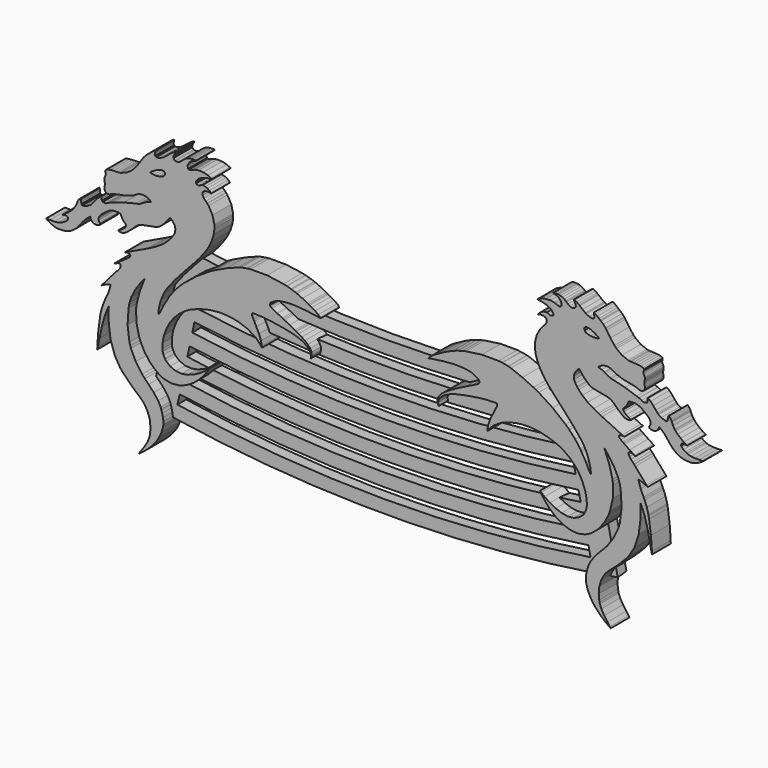
from build123d import *

# Parameters (mm, degrees)
F1_DEPTH               = 3.175
DRAFT_F1_DRAFTED_ANGLE = -3
F3_DEPTH               = 6.35


# Not quite as in the source:
# - an extrude with a draft is written as a straight extrude whose walls are then drafted
# - ends of sketch curves that miss each other by under 0.0002 mm in the source are joined
# - a pattern or mirror of a feature is missing from the dataset's text; its kind, count and spacing are read off the source's solid


with BuildPart() as f1:
    # F0 (on Front) → F1 (new body)
    with BuildSketch(Plane.XZ):
        with BuildLine():
            ThreePointArc((54.301977702, 4.5850323172), (0, 0.5241036), (-54.301977702, 4.5850323172))
            Line((-54.301977702, 4.5850323172), (-63.0060462, -35.368103))
            ThreePointArc((-63.0060462, -35.368103), (0, -40.7508964), (63.0060498531, -35.3681242237))
            Line((63.0060498531, -35.3681242237), (54.301977702, 4.5850323172))
        make_face()
        with BuildLine():
            Line((-56.045319226, -33.2484517718), (-55.3915362015, -30.2474846268))
            ThreePointArc((-55.3915362015, -30.2474846268), (1.30253e-05, -34.4009011827), (55.391562695, -30.2474905326))
            Line((55.391562695, -30.2474905326), (56.0453444328, -33.2484517718))
            ThreePointArc((56.0453444328, -33.2484517718), (1.26034e-05, -37.5759051845), (-56.045319226, -33.2484517718))
        make_face(mode=Mode.SUBTRACT)
        with BuildLine():
            Line((-54.7066751621, -27.1038644939), (-54.0516224279, -24.097069181))
            ThreePointArc((-54.0516224279, -24.097069181), (1.26819e-05, -28.0509044403), (54.051647871, -24.0970702655))
            Line((54.051647871, -24.0970702655), (54.7067017769, -27.103870957))
            ThreePointArc((54.7067017769, -27.103870957), (1.30639e-05, -31.2259008161), (-54.7066751621, -27.1038644939))
        make_face(mode=Mode.SUBTRACT)
        with BuildLine():
            Line((-53.366962814, -20.954373623), (-52.7106531283, -17.9418087047))
            ThreePointArc((-52.7106531283, -17.9418087047), (1.26417e-05, -21.7009048215), (52.710678449, -17.9418092272))
            Line((52.710678449, -17.9418092272), (53.3669877397, -20.9543723325))
            ThreePointArc((53.3669877397, -20.9543723325), (1.25103e-05, -24.875906068), (-53.366962814, -20.954373623))
        make_face(mode=Mode.SUBTRACT)
        with BuildLine():
            Line((-52.0261755137, -14.7999485521), (-51.3686274817, -11.7816994289))
            ThreePointArc((-51.3686274817, -11.7816994289), (1.29118e-05, -15.3509022613), (51.3686535941, -11.7817035856))
            Line((51.3686535941, -11.7817035856), (52.0262007398, -14.7999486408))
            ThreePointArc((52.0262007398, -14.7999486408), (1.26099e-05, -18.525905123), (-52.0261755137, -14.7999485521))
        make_face(mode=Mode.SUBTRACT)
        with BuildLine():
            Line((-50.6843154191, -8.6405991862), (-50.0255472782, -5.6167495712))
            ThreePointArc((-50.0255472782, -5.6167495712), (1.27309e-05, -9.0009039764), (50.0255728549, -5.6167512685))
            Line((50.0255728549, -5.6167512685), (50.6843403575, -8.640597954))
            ThreePointArc((50.6843403575, -8.640597954), (1.25122e-05, -12.1759060495), (-50.6843154191, -8.6405991862))
        make_face(mode=Mode.SUBTRACT)
        with BuildLine():
            Line((-49.3413790575, -2.4763095853), (-48.6814090209, 0.5530569207))
            ThreePointArc((-48.6814090209, 0.5530569207), (1.28477e-05, -2.6509028695), (48.6814349279, 0.5530537068))
            Line((48.6814349279, 0.5530537068), (49.3414053122, -2.4763143953))
            ThreePointArc((49.3414053122, -2.4763143953), (1.29641e-05, -5.8259017661), (-49.3413790575, -2.4763095853))
        make_face(mode=Mode.SUBTRACT)
    extrude(amount=F1_DEPTH)

    # draft_F1_drafted
    draft_f1_drafted_walls = [f1.faces().sort_by_distance(p)[0] for p in [
        (9.199e-07, -2.1166666667, -40.7508964),
        (58.6540137775, -2.1166666667, -15.3915459532),
        (0, -2.1166666667, 0.5241036),
        (-58.654011951, -2.1166666667, -15.3915353414),
        (55.7184535639, -2.1166666667, -31.7479711522),
        (1.26034e-05, -2.1166666667, -37.5759051845),
        (-55.7184277137, -2.1166666667, -31.7479681993),
        (1.30253e-05, -2.1166666667, -34.4009011827),
        (-54.379148795, -2.1166666667, -25.6004668374),
        (1.26819e-05, -2.1166666667, -28.0509044403),
        (54.379174824, -2.1166666667, -25.6004706112),
        (1.30639e-05, -2.1166666667, -31.2259008161),
        (-53.0388079711, -2.1166666667, -19.4480911639),
        (1.26417e-05, -2.1166666667, -21.7009048215),
        (53.0388330943, -2.1166666667, -19.4480907798),
        (1.25103e-05, -2.1166666667, -24.875906068),
        (-51.6974014977, -2.1166666667, -13.2908239905),
        (1.29118e-05, -2.1166666667, -15.3509022613),
        (51.697427167, -2.1166666667, -13.2908261132),
        (1.26099e-05, -2.1166666667, -18.525905123),
        (-50.3549313487, -2.1166666667, -7.1286743787),
        (1.27309e-05, -2.1166666667, -9.0009039764),
        (50.3549566062, -2.1166666667, -7.1286746113),
        (1.25122e-05, -2.1166666667, -12.1759060495),
        (-49.0113940392, -2.1166666667, -0.9616263323),
        (1.28477e-05, -2.1166666667, -2.6509028695),
        (49.0114201201, -2.1166666667, -0.9616303443),
        (1.29641e-05, -2.1166666667, -5.8259017661),
    ]]
    draft(draft_f1_drafted_walls, neutral_plane=Plane.XZ, angle=DRAFT_F1_DRAFTED_ANGLE)

    # F2 (on Front) → F3 (join)
    with BuildSketch(Plane.XZ):
        with BuildLine():
            Line((68.4158652, 8.8282272), (68.6661822, 9.411335))
            ThreePointArc((68.6661822, 9.411335), (70.4497514451, 9.5479214977), (72.1365475574, 8.9525417468))
            Line((72.1365475574, 8.9525417468), (72.3567006, 8.7865712))
            Line((72.3567006, 8.7865712), (72.4553542, 8.712581))
            Line((72.4553542, 8.712581), (72.7564712, 8.4946236))
            Line((72.7564712, 8.4946236), (73.2147634, 8.1538318))
            Line((73.2147634, 8.1538318), (73.6795326, 7.7712062))
            Line((73.6795326, 7.7712062), (74.1016552, 7.3527666))
            Line((74.1016552, 7.3527666), (74.4297724, 6.9043296))
            Line((74.4297724, 6.9043296), (74.6142526, 6.4323722))
            Line((74.6142526, 6.4323722), (74.6052356, 5.9422792))
            Line((74.6052356, 5.9422792), (74.4351064, 5.5500016))
            Line((74.4351064, 5.5500016), (74.3511086, 5.4405022))
            Line((74.3511086, 5.4405022), (74.3087922, 5.38734))
            Line((74.3087922, 5.38734), (74.2272836, 5.1891946))
            Line((74.2272836, 5.1891946), (74.2681268, 4.9929034))
            Line((74.2681268, 4.9929034), (74.4351064, 4.8472598))
            Line((74.4351064, 4.8472598), (74.6910622, 4.7470822))
            Line((74.6910622, 4.7470822), (74.9957098, 4.6882812))
            Line((74.9957098, 4.6882812), (75.3129812, 4.665599))
            Line((75.3129812, 4.665599), (75.602465, 4.6737778))
            Line((75.602465, 4.6737778), (75.7734324, 4.6935898))
            Line((75.7734324, 4.6935898), (75.8284234, 4.707255))
            Line((75.8284234, 4.707255), (75.932411, 4.734433))
            Line((75.932411, 4.734433), (76.2253746, 4.902581))
            Line((76.2253746, 4.902581), (76.5554984, 5.235194))
            Line((76.5554984, 5.235194), (76.7814568, 5.6511444))
            Line((76.7814568, 5.6511444), (76.8672834, 5.9849258))
            Line((76.8672834, 5.9849258), (76.8699504, 6.0960762))
            Line((76.8699504, 6.0960762), (77.0734298, 5.9551062))
            Line((77.0734298, 5.9551062), (77.6601952, 5.495671))
            Line((77.6601952, 5.495671), (78.3445982, 4.8590708))
            Line((78.3445982, 4.8590708), (78.957678, 4.1556686))
            Line((78.957678, 4.1556686), (79.4008064, 3.5590734))
            Line((79.4008064, 3.5590734), (79.537941, 3.3527746))
            Line((79.537941, 3.3527746), (79.6972498, 3.1141416))
            Line((79.6972498, 3.1141416), (80.6871386, 2.0456144))
            Line((80.6871386, 2.0456144), (81.8571642, 1.1738864))
            Line((81.8571642, 1.1738864), (82.1066176, 1.0330688))
            Line((82.1066176, 1.0330688), (82.3129164, 0.9172448))
            Line((82.3129164, 0.9172448), (82.977355, 0.6477762))
            Line((82.977355, 0.6477762), (83.837907, 0.4498086))
            Line((83.837907, 0.4498086), (84.7266276, 0.3784854))
            Line((84.7266276, 0.3784854), (85.4408502, 0.367665))
            Line((85.4408502, 0.367665), (85.6798388, 0.367665))
            Line((85.6798388, 0.367665), (85.8596454, 0.367665))
            Line((85.8596454, 0.367665), (86.3993954, 0.5149596))
            Line((86.3993954, 0.5149596), (87.341456, 0.8784336))
            Line((87.341456, 0.8784336), (88.2373394, 1.341374))
            Line((88.2373394, 1.341374), (88.7067822, 1.6533114))
            Line((88.7067822, 1.6533114), (88.8187708, 1.7851374))
            Line((88.8187708, 1.7851374), (88.5521216, 1.792478))
            Line((88.5521216, 1.792478), (87.7500658, 1.7734788))
            Line((87.7500658, 1.7734788), (86.6028748, 1.7634712))
            Line((86.6028748, 1.7634712), (85.4798646, 1.8737834))
            Line((85.4798646, 1.8737834), (84.7096096, 2.0934426))
            Line((84.7096096, 2.0934426), (84.4836512, 2.220087))
            Line((84.4836512, 2.220087), (84.376006, 2.2807422))
            Line((84.376006, 2.2807422), (84.0531974, 2.4558752))
            Line((84.0531974, 2.4558752), (83.5351136, 2.7788362))
            Line((83.5351136, 2.7788362), (83.0911724, 3.170301))
            Line((83.0911724, 3.170301), (82.8950082, 3.495929))
            Line((82.8950082, 3.495929), (82.8878454, 3.6079176))
            Line((82.8878454, 3.6079176), (82.8825114, 3.6847272))
            Line((82.8825114, 3.6847272), (82.9176904, 3.9180262))
            Line((82.9176904, 3.9180262), (83.0433442, 4.1068498))
            Line((83.0433442, 4.1068498), (83.2403212, 4.1993312))
            Line((83.2403212, 4.1993312), (83.4854566, 4.2181526))
            Line((83.4854566, 4.2181526), (83.7547474, 4.188333))
            Line((83.7547474, 4.188333), (84.0260448, 4.133342))
            Line((84.0260448, 4.133342), (84.2746854, 4.076192))
            Line((84.2746854, 4.076192), (84.427314, 4.0465248))
            Line((84.427314, 4.0465248), (84.4789776, 4.0418512))
            Line((84.4789776, 4.0418512), (84.257515, 4.1901618))
            Line((84.257515, 4.1901618), (83.59394, 4.6322742))
            Line((83.59394, 4.6322742), (82.7385442, 5.2470304))
            Line((82.7385442, 5.2470304), (81.9439814, 5.9277758))
            Line((81.9439814, 5.9277758), (81.4005484, 6.5073784))
            Line((81.4005484, 6.5073784), (81.2432208, 6.7171824))
            Line((81.2432208, 6.7171824), (81.1339246, 6.862826))
            Line((81.1339246, 6.862826), (80.7036232, 7.5662282))
            Line((80.7036232, 7.5662282), (80.3853358, 8.321802))
            Line((80.3853358, 8.321802), (80.3328594, 8.492617))
            Line((80.3328594, 8.492617), (80.320007, 8.5324442))
            Line((80.320007, 8.5324442), (80.2668448, 8.6465918))
            Line((80.2668448, 8.6465918), (80.1520368, 8.8535764))
            Line((80.1520368, 8.8535764), (80.0045644, 9.0797126))
            Line((80.0045644, 9.0797126), (79.8419028, 9.2903548))
            Line((79.8419028, 9.2903548), (79.6790888, 9.4501716))
            Line((79.6790888, 9.4501716), (79.532607, 9.5251524))
            Line((79.532607, 9.5251524), (79.4206438, 9.479153))
            Line((79.4206438, 9.479153), (79.3634684, 9.3300042))
            Line((79.3634684, 9.3300042), (79.3581344, 9.2785184))
            Line((79.3581344, 9.2785184), (79.3438088, 9.1528646))
            Line((79.3438088, 9.1528646), (79.3309818, 8.7704168))
            Line((79.3309818, 8.7704168), (79.2659832, 8.3238086))
            Line((79.2659832, 8.3238086), (79.0208478, 8.0633316))
            Line((79.0208478, 8.0633316), (78.58506, 8.0715104))
            Line((78.58506, 8.0715104), (78.4530816, 8.1131664))
            Line((78.4530816, 8.1131664), (78.3029422, 8.1609946))
            Line((78.3029422, 8.1609946), (77.496543, 8.4711286))
            Line((77.496543, 8.4711286), (76.7696458, 8.9150698))
            Line((76.7696458, 8.9150698), (76.6603242, 9.0298778))
            Line((76.6603242, 9.0298778), (76.4919984, 9.2053664))
            Line((76.4919984, 9.2053664), (76.0292358, 9.768459))
            Line((76.0292358, 9.768459), (75.336654, 10.6211878))
            Line((75.336654, 10.6211878), (74.5980728, 11.405743))
            Line((74.5980728, 11.405743), (74.0409746, 11.846179))
            Line((74.0409746, 11.846179), (73.8321866, 11.9401844))
            Line((73.8321866, 11.9401844), (73.8276908, 11.7873526))
            Line((73.8276908, 11.7873526), (73.8241856, 11.327257))
            Line((73.8241856, 11.327257), (73.751694, 10.9139736))
            Line((73.751694, 10.9139736), (73.4887278, 10.6825034))
            Line((73.4887278, 10.6825034), (73.0519494, 10.6093514))
            Line((73.0519494, 10.6093514), (72.9072964, 10.6093514))
            Line((72.9072964, 10.6093514), (72.7184982, 10.6093514))
            Line((72.7184982, 10.6093514), (72.1513924, 10.8426504))
            Line((72.1513924, 10.8426504), (71.5494632, 11.1581184))
            Line((71.5494632, 11.1581184), (71.423657, 11.1997744))
            Line((71.423657, 11.1997744), (70.809739, 11.4050826))
            Line((70.809739, 11.4050826), (67.7077894, 12.4300996))
            Line((67.7077894, 12.4300996), (64.5488676, 13.229336))
            Line((64.5488676, 13.229336), (63.9069588, 13.3208268))
            Line((63.9069588, 13.3208268), (63.8001264, 13.3359906))
            Line((63.8001264, 13.3359906), (63.4918466, 13.4644892))
            Line((63.4918466, 13.4644892), (63.0263916, 13.7292842))
            Line((63.0263916, 13.7292842), (62.5634512, 14.0232384))
            Line((62.5634512, 14.0232384), (62.2596672, 14.2058898))
            Line((62.2596672, 14.2058898), (62.1538508, 14.2555468))
            Line((62.1538508, 14.2555468), (62.0300258, 14.313535))
            Line((62.0300258, 14.313535), (61.405262, 14.6218402))
            Line((61.405262, 14.6218402), (60.7561904, 14.8551392))
            Line((60.7561904, 14.8551392), (60.6213672, 14.8759672))
            Line((60.6213672, 14.8759672), (60.5907094, 14.8803106))
            Line((60.5907094, 14.8803106), (60.505721, 14.938121))
            Line((60.505721, 14.938121), (60.5498662, 15.0476204))
            Line((60.5498662, 15.0476204), (60.7118674, 15.1885904))
            Line((60.7118674, 15.1885904), (60.9486716, 15.3440638))
            Line((60.9486716, 15.3440638), (61.219969, 15.4978862))
            Line((61.219969, 15.4978862), (61.4812588, 15.6325316))
            Line((61.4812588, 15.6325316), (61.6927392, 15.7311852))
            Line((61.6927392, 15.7311852), (61.780547, 15.7700218))
            Line((61.780547, 15.7700218), (61.8113826, 15.7771846))
            Line((61.8113826, 15.7771846), (61.9750348, 15.8188406))
            Line((61.9750348, 15.8188406), (62.7324374, 15.9056578))
            Line((62.7324374, 15.9056578), (63.489332, 15.8188406))
            Line((63.489332, 15.8188406), (63.6536446, 15.7728412))
            Line((63.6536446, 15.7728412), (63.8048, 15.7301946))
            Line((63.8048, 15.7301946), (64.4963658, 15.360396))
            Line((64.4963658, 15.360396), (65.1771112, 14.953615))
            Line((65.1771112, 14.953615), (65.323593, 14.8929598))
            Line((65.323593, 14.8929598), (65.4764248, 14.8296376))
            Line((65.4764248, 14.8296376), (67.0170618, 14.2673832))
            Line((67.0170618, 14.2673832), (67.1780216, 14.2257272))
            Line((67.1780216, 14.2257272), (67.4753286, 14.1488922))
            Line((67.4753286, 14.1488922), (69.0124604, 13.8775948))
            Line((69.0124604, 13.8775948), (70.5331076, 13.5494776))
            Line((70.5331076, 13.5494776), (70.8234042, 13.4446518))
            Line((70.8234042, 13.4446518), (70.9318876, 13.4056628))
            Line((70.9318876, 13.4056628), (71.250175, 13.2628386))
            Line((71.250175, 13.2628386), (71.701279, 13.0893566))
            Line((71.701279, 13.0893566), (72.1614, 13.0348736))
            Line((72.1614, 13.0348736), (72.5221816, 13.1435094))
            Line((72.5221816, 13.1435094), (72.6171776, 13.2131816))
            Line((72.6171776, 13.2131816), (72.7001594, 13.2756656))
            Line((72.7001594, 13.2756656), (72.896476, 13.534136))
            Line((72.896476, 13.534136), (73.0402908, 13.9364212))
            Line((73.0402908, 13.9364212), (73.0611188, 14.365859))
            Line((73.0611188, 14.365859), (73.0084392, 14.670659))
            Line((73.0084392, 14.670659), (72.9724474, 14.764639))
            Line((72.9724474, 14.764639), (72.9326202, 14.867636))
            Line((72.9326202, 14.867636), (72.9101412, 15.214092))
            Line((72.9101412, 15.214092), (72.9814644, 15.673197))
            Line((72.9814644, 15.673197), (73.0682816, 16.1299652))
            Line((73.0682816, 16.1299652), (73.0772732, 16.4652706))
            Line((73.0772732, 16.4652706), (73.0511112, 16.5692582))
            Line((73.0511112, 16.5692582), (73.0249492, 16.6722298))
            Line((73.0249492, 16.6722298), (72.891142, 16.9670222))
            Line((72.891142, 16.9670222), (72.725661, 17.2871638))
            Line((72.725661, 17.2871638), (72.656827, 17.6316132))
            Line((72.656827, 17.6316132), (72.7391484, 17.9940712))
            Line((72.7391484, 17.9940712), (72.7906342, 18.1025546))
            Line((72.7906342, 18.1025546), (72.8268038, 18.1803802))
            Line((72.8268038, 18.1803802), (72.8042994, 18.4749948))
            Line((72.8042994, 18.4749948), (72.5013536, 18.735294))
            Line((72.5013536, 18.735294), (71.968741, 18.9046104))
            Line((71.968741, 18.9046104), (71.2953362, 19.0041022))
            Line((71.2953362, 19.0041022), (70.5682612, 19.0545974))
            Line((70.5682612, 19.0545974), (69.8758572, 19.0780924))
            Line((69.8758572, 19.0780924), (69.3052462, 19.0944246))
            Line((69.3052462, 19.0944246), (69.0332884, 19.108928))
            Line((69.0332884, 19.108928), (68.9464712, 19.1260984))
            Line((68.9464712, 19.1260984), (68.571364, 19.2037462))
            Line((68.571364, 19.2037462), (66.8724088, 19.8726552))
            Line((66.8724088, 19.8726552), (65.3895822, 20.9478626))
            Line((65.3895822, 20.9478626), (65.1237966, 21.227161))
            Line((65.1237966, 21.227161), (64.8688314, 21.4947754))
            Line((64.8688314, 21.4947754), (63.7569718, 22.9667562))
            Line((63.7569718, 22.9667562), (62.7244364, 24.501729))
            Line((62.7244364, 24.501729), (62.5101366, 24.8003568))
            Line((62.5101366, 24.8003568), (62.4124736, 24.935688))
            Line((62.4124736, 24.935688), (61.8373922, 25.567767))
            Line((61.8373922, 25.567767), (61.1919528, 26.129361))
            Line((61.1919528, 26.129361), (61.059822, 26.2295132))
            Line((61.059822, 26.2295132), (60.9531674, 26.3101582))
            Line((60.9531674, 26.3101582), (60.6522028, 26.5741404))
            Line((60.6522028, 26.5741404), (60.1910912, 26.9774162))
            Line((60.1910912, 26.9774162), (59.710828, 27.3335496))
            Line((59.710828, 27.3335496), (59.3712046, 27.5106892))
            Line((59.3712046, 27.5106892), (59.250707, 27.5341842))
            Line((59.250707, 27.5341842), (59.2470494, 27.4293584))
            Line((59.2470494, 27.4293584), (59.3213698, 27.1120616))
            Line((59.3213698, 27.1120616), (59.4251796, 26.6292838))
            Line((59.4251796, 26.6292838), (59.3647022, 26.2205216))
            Line((59.3647022, 26.2205216), (59.051063, 26.0298692))
            Line((59.051063, 26.0298692), (58.9434178, 26.0217158))
            Line((58.9434178, 26.0217158), (58.7689452, 26.0098794))
            Line((58.7689452, 26.0098794), (57.9815452, 26.1716774))
            Line((57.9815452, 26.1716774), (57.253632, 26.5442954))
            Line((57.253632, 26.5442954), (57.1098172, 26.6372848))
            Line((57.1098172, 26.6372848), (56.952515, 26.7387832))
            Line((56.952515, 26.7387832), (56.2157626, 27.3118834))
            Line((56.2157626, 27.3118834), (55.4950376, 27.9066244))
            Line((55.4950376, 27.9066244), (55.3458888, 28.0179526))
            Line((55.3458888, 28.0179526), (55.2653962, 28.0786078))
            Line((55.2653962, 28.0786078), (55.0149268, 28.2612592))
            Line((55.0149268, 28.2612592), (54.5766498, 28.5530544))
            Line((54.5766498, 28.5530544), (54.1308544, 28.78201))
            Line((54.1308544, 28.78201), (53.8603952, 28.8570162))
            Line((53.8603952, 28.8570162), (53.7827474, 28.8361882))
            Line((53.7827474, 28.8361882), (53.8505654, 28.7015428))
            Line((53.8505654, 28.7015428), (54.0971994, 28.3162502))
            Line((54.0971994, 28.3162502), (54.3731704, 27.8026368))
            Line((54.3731704, 27.8026368), (54.3893248, 27.3137122))
            Line((54.3893248, 27.3137122), (54.0630364, 26.9419324))
            Line((54.0630364, 26.9419324), (53.9274004, 26.868755))
            Line((53.9274004, 26.868755), (53.7979112, 26.8000988))
            Line((53.7979112, 26.8000988), (53.3259792, 26.7477748))
            Line((53.3259792, 26.7477748), (52.7620484, 26.9474188))
            Line((52.7620484, 26.9474188), (52.2456156, 27.3255486))
            Line((52.2456156, 27.3255486), (51.9013186, 27.6346666))
            Line((51.9013186, 27.6346666), (51.7865106, 27.7368254))
            Line((51.7865106, 27.7368254), (51.6670036, 27.842464))
            Line((51.6670036, 27.842464), (51.2874006, 28.1327606))
            Line((51.2874006, 28.1327606), (50.7837948, 28.4220666))
            Line((50.7837948, 28.4220666), (50.235866, 28.6183832))
            Line((50.235866, 28.6183832), (49.7674138, 28.7150302))
            Line((49.7674138, 28.7150302), (49.6102894, 28.7322006))
            Line((49.6102894, 28.7322006), (49.5577876, 28.7385252))
            Line((49.5577876, 28.7385252), (49.3234726, 28.7556956))
            Line((49.3234726, 28.7556956), (48.8933744, 28.7711896))
            Line((48.8933744, 28.7711896), (48.4900986, 28.7493456))
            Line((48.4900986, 28.7493456), (48.2984556, 28.698698))
            Line((48.2984556, 28.698698), (48.285781, 28.6625284))
            Line((48.285781, 28.6625284), (48.2794564, 28.6482028))
            Line((48.2794564, 28.6482028), (48.3805992, 28.5577026))
            Line((48.3805992, 28.5577026), (48.6518966, 28.4708854))
            Line((48.6518966, 28.4708854), (48.9501942, 28.4102302))
            Line((48.9501942, 28.4102302), (49.1066836, 28.3850588))
            Line((49.1066836, 28.3850588), (49.1300008, 28.3822394))
            Line((49.1300008, 28.3822394), (49.2484918, 28.3695648))
            Line((49.2484918, 28.3695648), (49.5876072, 28.1769312))
            Line((49.5876072, 28.1769312), (50.04689, 27.7439882))
            Line((50.04689, 27.7439882), (50.4005088, 27.2187162))
            Line((50.4005088, 27.2187162), (50.542317, 26.856944))
            Line((50.542317, 26.856944), (50.542317, 26.7359384))
            Line((50.542317, 26.7359384), (50.542317, 26.6372848))
            Line((50.542317, 26.6372848), (50.5024898, 26.341832))
            Line((50.5024898, 26.341832), (50.3905012, 26.0966966))
            Line((50.3905012, 26.0966966), (50.2170446, 25.9747004))
            Line((50.2170446, 25.9747004), (49.9909084, 25.9538724))
            Line((49.9909084, 25.9538724), (49.7224304, 26.0080506))
            Line((49.7224304, 26.0080506), (49.4221262, 26.112851))
            Line((49.4221262, 26.112851), (49.1005114, 26.2460232))
            Line((49.1005114, 26.2460232), (48.850042, 26.3489948))
            Line((48.850042, 26.3489948), (48.76673, 26.3806686))
            Line((48.76673, 26.3806686), (48.4872538, 26.4873232))
            Line((48.4872538, 26.4873232), (47.5823788, 26.635456))
            Line((47.5823788, 26.635456), (46.3065368, 26.5848084))
            Line((46.3065368, 26.5848084), (45.063537, 26.264997))
            Line((45.063537, 26.264997), (44.2253116, 25.8813808))
            Line((44.2253116, 25.8813808), (43.9749946, 25.7115818))
            Line((43.9749946, 25.7115818), (44.2779658, 25.682575))
            Line((44.2779658, 25.682575), (45.1828408, 25.5532636))
            Line((45.1828408, 25.5532636), (46.532673, 25.2069854))
            Line((46.532673, 25.2069854), (47.6971868, 24.57323))
            Line((47.6971868, 24.57323), (48.285781, 23.8309912))
            Line((48.285781, 23.8309912), (48.3497636, 23.552531))
            Line((48.3497636, 23.552531), (48.362616, 23.4956858))
            Line((48.362616, 23.4956858), (48.2894386, 23.2965498))
            Line((48.2894386, 23.2965498), (48.047148, 23.1257348))
            Line((48.047148, 23.1257348), (47.737014, 23.0354124))
            Line((47.737014, 23.0354124), (47.5388686, 23.0137462))
            Line((47.5388686, 23.0137462), (47.4757242, 23.0209344))
            Line((47.4757242, 23.0209344), (47.3907358, 23.0309166))
            Line((47.3907358, 23.0309166), (47.001938, 23.2595674))
            Line((47.001938, 23.2595674), (46.5814918, 23.4566968))
            Line((46.5814918, 23.4566968), (46.4811872, 23.4501944))
            Line((46.4811872, 23.4501944), (46.2975452, 23.4395264))
            Line((46.2975452, 23.4395264), (45.7524358, 23.3482134))
            Line((45.7524358, 23.3482134), (45.1773544, 23.124922))
            Line((45.1773544, 23.124922), (44.6782444, 22.7559616))
            Line((44.6782444, 22.7559616), (44.2941202, 22.3536764))
            Line((44.2941202, 22.3536764), (44.1774834, 22.2108522))
            Line((44.1774834, 22.2108522), (44.3211204, 22.2615252))
            Line((44.3211204, 22.2615252), (44.776898, 22.3465136))
            Line((44.776898, 22.3465136), (45.49648, 22.3601788))
            Line((45.49648, 22.3601788), (46.1410558, 22.1620334))
            Line((46.1410558, 22.1620334), (46.4791806, 21.7985848))
            Line((46.4791806, 21.7985848), (46.5146644, 21.657437))
            Line((46.5146644, 21.657437), (46.5516722, 21.5092788))
            Line((46.5516722, 21.5092788), (46.4791806, 21.0165188))
            Line((46.4791806, 21.0165188), (46.1395572, 20.4469238))
            Line((46.1395572, 20.4469238), (45.6576176, 19.9298306))
            Line((45.6576176, 19.9298306), (45.301154, 19.5735194))
            Line((45.301154, 19.5735194), (45.193839, 19.445224))
            Line((45.193839, 19.445224), (44.8960494, 19.0944246))
            Line((44.8960494, 19.0944246), (43.829351, 17.213834))
            Line((43.829351, 17.213834), (43.3347368, 15.1082756))
            Line((43.3347368, 15.1082756), (43.3240942, 14.6453352))
            Line((43.3240942, 14.6453352), (43.3122578, 14.1642338))
            Line((43.3122578, 14.1642338), (43.5012338, 12.7140716))
            Line((43.5012338, 12.7140716), (44.0716416, 10.8659676))
            Line((44.0716416, 10.8659676), (44.9567046, 9.0987118))
            Line((44.9567046, 9.0987118), (46.078902, 7.411593))
            Line((46.078902, 7.411593), (47.3562426, 5.8012838))
            Line((47.3562426, 5.8012838), (48.7115612, 4.2679874))
            Line((48.7115612, 4.2679874), (50.0658892, 2.8086812))
            Line((50.0658892, 2.8086812), (51.0260854, 1.7734788))
            Line((51.0260854, 1.7734788), (51.3397246, 1.4226794))
            Line((51.3397246, 1.4226794), (51.763676, 0.9489186))
            Line((51.763676, 0.9489186), (53.8369002, -1.3692886))
            Line((53.8369002, -1.3692886), (55.78983, -3.7839904))
            Line((55.78983, -3.7839904), (56.1551074, -4.307586))
            Line((56.1551074, -4.307586), (56.403748, -4.663694))
            Line((56.403748, -4.663694), (57.0383162, -5.8128916))
            Line((57.0383162, -5.8128916), (57.778904, -7.565009))
            Line((57.778904, -7.565009), (58.2788268, -9.3914214))
            Line((58.2788268, -9.3914214), (58.4506578, -10.687939))
            Line((58.4506578, -10.687939), (58.4406502, -11.118215))
            Line((58.4406502, -11.118215), (58.325004, -11.0252256))
            Line((58.325004, -11.0252256), (58.0473566, -10.6615992))
            Line((58.0473566, -10.6615992), (57.7390768, -10.0785168))
            Line((57.7390768, -10.0785168), (57.4759328, -9.4610936))
            Line((57.4759328, -9.4610936), (57.2887856, -9.0351356))
            Line((57.2887856, -9.0351356), (57.2156336, -8.8994996))
            Line((57.2156336, -8.8994996), (57.1069978, -8.6988396))
            Line((57.1069978, -8.6988396), (55.951628, -6.7432682))
            Line((55.951628, -6.7432682), (55.8378106, -6.5471294))
            Line((55.8378106, -6.5471294), (55.6045116, -6.1438536))
            Line((55.6045116, -6.1438536), (54.2266886, -4.2415968))
            Line((54.2266886, -4.2415968), (52.6372328, -2.5119838))
            Line((52.6372328, -2.5119838), (52.298092, -2.194687))
            Line((52.298092, -2.194687), (51.6380222, -1.577086))
            Line((51.6380222, -1.577086), (48.135794, 1.2535408))
            Line((48.135794, 1.2535408), (44.3447932, 3.6828984))
            Line((44.3447932, 3.6828984), (43.5408832, 4.099687))
            Line((43.5408832, 4.099687), (42.9504602, 4.406138))
            Line((42.9504602, 4.406138), (39.95801, 5.8157872))
            Line((39.95801, 5.8157872), (36.8795808, 7.012813))
            Line((36.8795808, 7.012813), (36.2456476, 7.2134476))
            Line((36.2456476, 7.2134476), (36.0993436, 7.2604376))
            Line((36.0993436, 7.2604376), (34.5713812, 7.5299062))
            Line((34.5713812, 7.5299062), (34.41573, 7.5435714))
            Line((34.41573, 7.5435714), (33.5216754, 7.6592176))
            Line((33.5216754, 7.6592176), (29.0399724, 7.6735432))
            Line((29.0399724, 7.6735432), (24.6496078, 7.0534784))
            Line((24.6496078, 7.0534784), (23.8015526, 6.8519802))
            Line((23.8015526, 6.8519802), (23.6930692, 6.826504))
            Line((23.6930692, 6.826504), (22.625304, 6.5362074))
            Line((22.625304, 6.5362074), (22.5204274, 6.5028826))
            Line((22.5204274, 6.5028826), (22.4146618, 6.4702182))
            Line((22.4146618, 6.4702182), (21.3722204, 6.1059314))
            Line((21.3722204, 6.1059314), (21.2700362, 6.06425))
            Line((21.2700362, 6.06425), (20.9635344, 5.9432698))
            Line((20.9635344, 5.9432698), (19.5052188, 5.291201))
            Line((19.5052188, 5.291201), (18.088483, 4.5526198))
            Line((18.088483, 4.5526198), (17.8036982, 4.3881294))
            Line((17.8036982, 4.3881294), (17.5984662, 4.2704766))
            Line((17.5984662, 4.2704766), (16.971899, 3.9360348))
            Line((16.971899, 3.9360348), (16.0633156, 3.4224214))
            Line((16.0633156, 3.4224214), (15.2269952, 2.8276804))
            Line((15.2269952, 2.8276804), (14.728825, 2.3277322))
            Line((14.728825, 2.3277322), (14.6103848, 2.1324316))
            Line((14.6103848, 2.1324316), (15.2504902, 2.246249))
            Line((15.2504902, 2.246249), (18.498058, 2.7081988))
            Line((18.498058, 2.7081988), (21.4382096, 2.9424884))
            Line((21.4382096, 2.9424884), (22.4182686, 2.9424884))
            Line((22.4182686, 2.9424884), (22.8739192, 2.9424884))
            Line((22.8739192, 2.9424884), (24.2409472, 2.8638246))
            Line((24.2409472, 2.8638246), (25.748107, 2.629535))
            Line((25.748107, 2.629535), (26.037413, 2.5520396))
            Line((26.037413, 2.5520396), (26.1178802, 2.5312116))
            Line((26.1178802, 2.5312116), (26.3547606, 2.4478996))
            Line((26.3547606, 2.4478996), (26.7887196, 2.2707346))
            Line((26.7887196, 2.2707346), (27.2715228, 2.033778))
            Line((27.2715228, 2.033778), (27.7353268, 1.7509744))
            Line((27.7353268, 1.7509744), (28.1105356, 1.4351762))
            Line((28.1105356, 1.4351762), (28.33116, 1.1008868))
            Line((28.33116, 1.1008868), (28.3275278, 0.7599426))
            Line((28.3275278, 0.7599426), (28.120467, 0.4894834))
            Line((28.120467, 0.4894834), (28.0327862, 0.4273042))
            Line((28.0327862, 0.4273042), (27.7796244, 0.2510028))
            Line((27.7796244, 0.2510028), (26.3701276, -0.4760722))
            Line((26.3701276, -0.4760722), (24.920829, -1.147826))
            Line((24.920829, -1.147826), (24.6486934, -1.2977876))
            Line((24.6486934, -1.2977876), (24.372951, -1.448943))
            Line((24.372951, -1.448943), (22.9580186, -2.168525))
            Line((22.9580186, -2.168525), (21.5557354, -2.906268))
            Line((21.5557354, -2.906268), (21.287232, -3.0672278))
            Line((21.287232, -3.0672278), (21.1072984, -3.1738824))
            Line((21.1072984, -3.1738824), (20.5639416, -3.4875216))
            Line((20.5639416, -3.4875216), (19.730339, -3.9857934))
            Line((19.730339, -3.9857934), (18.8741558, -4.5578776))
            Line((18.8741558, -4.5578776), (18.0830728, -5.1999642))
            Line((18.0830728, -5.1999642), (17.4456598, -5.905881))
            Line((17.4456598, -5.905881), (17.0478704, -6.6717672))
            Line((17.0478704, -6.6717672), (16.9800524, -7.4946764))
            Line((16.9800524, -7.4946764), (17.2024548, -8.17626))
            Line((17.2024548, -8.17626), (17.3290484, -8.3697318))
            Line((17.3290484, -8.3697318), (17.2557948, -8.181594))
            Line((17.2557948, -8.181594), (17.1798488, -7.5643232))
            Line((17.1798488, -7.5643232), (17.3480222, -6.840093))
            Line((17.3480222, -6.840093), (17.7675286, -6.1961776))
            Line((17.7675286, -6.1961776), (18.3723788, -5.6339232))
            Line((18.3723788, -5.6339232), (19.0956692, -5.1536346))
            Line((19.0956692, -5.1536346), (19.8722996, -4.7541942))
            Line((19.8722996, -4.7541942), (20.6362808, -4.437888))
            Line((20.6362808, -4.437888), (21.1489036, -4.2567606))
            Line((21.1489036, -4.2567606), (21.3215728, -4.2035984))
            Line((21.3215728, -4.2035984), (21.8559126, -4.0381174))
            Line((21.8559126, -4.0381174), (24.6098314, -3.448685))
            Line((24.6098314, -3.448685), (27.3962876, -3.0074108))
            Line((27.3962876, -3.0074108), (27.9477978, -2.9160978))
            Line((27.9477978, -2.9160978), (28.2244546, -2.8699206))
            Line((28.2244546, -2.8699206), (30.4575718, -2.6412952))
            Line((30.4575718, -2.6412952), (31.2947812, -2.6412952))
            Line((31.2947812, -2.6412952), (31.3824366, -2.6412952))
            Line((31.3824366, -2.6412952), (31.6474094, -2.619629))
            Line((31.6474094, -2.619629), (32.1953382, -2.5861264))
            Line((32.1953382, -2.5861264), (32.7359264, -2.5871424))
            Line((32.7359264, -2.5871424), (33.014412, -2.6241248))
            Line((33.014412, -2.6241248), (33.0687172, -2.670302))
            Line((33.0687172, -2.670302), (33.1183996, -2.7134566))
            Line((33.1183996, -2.7134566), (33.1698854, -2.9614114))
            Line((33.1698854, -2.9614114), (33.0623926, -3.349371))
            Line((33.0623926, -3.349371), (32.8652632, -3.7416486))
            Line((32.8652632, -3.7416486), (32.7369424, -3.9702994))
            Line((32.7369424, -3.9702994), (32.7007728, -4.048125))
            Line((32.7007728, -4.048125), (32.5244714, -4.4203874))
            Line((32.5244714, -4.4203874), (31.9602104, -5.5235856))
            Line((31.9602104, -5.5235856), (31.2631328, -6.9459094))
            Line((31.2631328, -6.9459094), (30.7262022, -8.4185506))
            Line((30.7262022, -8.4185506), (30.4847244, -9.6380554))
            Line((30.4847244, -9.6380554), (30.464887, -10.0476812))
            Line((30.464887, -10.0476812), (30.7993542, -9.5179134))
            Line((30.7993542, -9.5179134), (32.1563492, -8.1519268))
            Line((32.1563492, -8.1519268), (34.3145618, -6.810248))
            Line((34.3145618, -6.810248), (36.7420906, -5.9431936))
            Line((36.7420906, -5.9431936), (38.6126736, -5.548757))
            Line((38.6126736, -5.548757), (39.2429492, -5.4737762))
            Line((39.2429492, -5.4737762), (39.9055082, -5.393436))
            Line((39.9055082, -5.393436), (41.916096, -5.3401214))
            Line((41.916096, -5.3401214), (44.4639446, -5.5869078))
            Line((44.4639446, -5.5869078), (46.957615, -6.18617))
            Line((46.957615, -6.18617), (48.8535472, -6.850761))
            Line((48.8535472, -6.850761), (49.4691416, -7.1120508))
            Line((49.4691416, -7.1120508), (49.9220744, -7.3038716))
            Line((49.9220744, -7.3038716), (51.2214114, -8.0244442))
            Line((51.2214114, -8.0244442), (52.805203, -9.1897962))
            Line((52.805203, -9.1897962), (54.190519, -10.5766108))
            Line((54.190519, -10.5766108), (55.0892472, -11.7394736))
            Line((55.0892472, -11.7394736), (55.3468794, -12.1535698))
            Line((55.3468794, -12.1535698), (55.5973488, -12.5566932))
            Line((55.5973488, -12.5566932), (56.2456076, -13.8305286))
            Line((56.2456076, -13.8305286), (56.947181, -15.6956252))
            Line((56.947181, -15.6956252), (57.3402968, -17.6350422))
            Line((57.3402968, -17.6350422), (57.3819528, -19.070701))
            Line((57.3819528, -19.070701), (57.3132966, -19.537299))
            Line((57.3132966, -19.537299), (57.2933068, -19.6682868))
            Line((57.2933068, -19.6682868), (57.0599824, -20.3990194))
            Line((57.0599824, -20.3990194), (56.6777124, -21.1610956))
            Line((56.6777124, -21.1610956), (56.583707, -21.3084156))
            Line((56.583707, -21.3084156), (56.3134256, -21.6493598))
            Line((56.3134256, -21.6493598), (55.2825412, -22.501098))
            Line((55.2825412, -22.501098), (53.8062424, -23.1248458))
            Line((53.8062424, -23.1248458), (52.2141196, -23.2631488))
            Line((52.2141196, -23.2631488), (50.5713238, -22.9982014))
            Line((50.5713238, -22.9982014), (48.9383578, -22.4159318))
            Line((48.9383578, -22.4159318), (47.3779088, -21.5985344))
            Line((47.3779088, -21.5985344), (45.9540864, -20.6304896))
            Line((45.9540864, -20.6304896), (45.0191886, -19.8692516))
            Line((45.0191886, -19.8692516), (44.7280792, -19.5951348))
            Line((44.7280792, -19.5951348), (44.9785486, -20.0627234))
            Line((44.9785486, -20.0627234), (45.879766, -21.3852252))
            Line((45.879766, -21.3852252), (47.3418916, -23.046182))
            Line((47.3418916, -23.046182), (49.0478572, -24.4818408))
            Line((49.0478572, -24.4818408), (50.9331214, -25.5948688))
            Line((50.9331214, -25.5948688), (52.9310092, -26.2882634))
            Line((52.9310092, -26.2882634), (54.977919, -26.466419))
            Line((54.977919, -26.466419), (57.0078362, -26.03246))
            Line((57.0078362, -26.03246), (58.5221334, -25.2412246))
            Line((58.5221334, -25.2412246), (58.9560924, -24.8896124))
            Line((58.9560924, -24.8896124), (59.0833972, -24.7974612))
            Line((59.0833972, -24.7974612), (60.2869, -23.759414))
            Line((60.2869, -23.759414), (60.3999046, -23.6455966))
            Line((60.3999046, -23.6455966), (60.7371912, -23.3011472))
            Line((60.7371912, -23.3011472), (62.1881662, -21.3652354))
            Line((62.1881662, -21.3652354), (63.2740416, -19.2651634))
            Line((63.2740416, -19.2651634), (63.4296674, -18.8392308))
            Line((63.4296674, -18.8392308), (63.6529842, -18.2226458))
            Line((63.6529842, -18.2226458), (64.3905494, -15.046706))
            Line((64.3905494, -15.046706), (64.4873742, -11.7889528))
            Line((64.4873742, -11.7889528), (64.3915654, -11.1318802))
            Line((64.3915654, -11.1318802), (64.2929118, -10.4609646))
            Line((64.2929118, -10.4609646), (63.4846584, -7.340854))
            Line((63.4846584, -7.340854), (62.3301522, -4.328414))
            Line((62.3301522, -4.328414), (62.0580166, -3.711829))
            Line((62.0580166, -3.711829), (62.4124736, -4.144772))
            Line((62.4124736, -4.144772), (63.4440184, -5.4747668))
            Line((63.4440184, -5.4747668), (64.728852, -7.3741788))
            Line((64.728852, -7.3741788), (65.7612096, -9.4059248))
            Line((65.7612096, -9.4059248), (66.297302, -11.016234))
            Line((66.297302, -11.016234), (66.3906216, -11.5674902))
            Line((66.3906216, -11.5674902), (66.5277816, -12.3803918))
            Line((66.5277816, -12.3803918), (66.7819086, -16.382873))
            Line((66.7819086, -16.382873), (66.2838146, -20.3502006))
            Line((66.2838146, -20.3502006), (66.0450038, -21.1465922))
            Line((66.0450038, -21.1465922), (65.873376, -21.7161872))
            Line((65.873376, -21.7161872), (64.5878566, -24.4248432))
            Line((64.5878566, -24.4248432), (62.8419114, -26.8741906))
            Line((62.8419114, -26.8741906), (62.4413026, -27.3144742))
            Line((62.4413026, -27.3144742), (62.1140236, -27.673427))
            Line((62.1140236, -27.673427), (61.0932992, -28.714954))
            Line((61.0932992, -28.714954), (59.7208102, -30.172279))
            Line((59.7208102, -30.172279), (58.524648, -31.7436754))
            Line((58.524648, -31.7436754), (57.8458838, -33.0320142))
            Line((57.8458838, -33.0320142), (57.707403, -33.4885792))
            Line((57.707403, -33.4885792), (57.6387468, -33.7137248))
            Line((57.6387468, -33.7137248), (57.439941, -34.3918032))
            Line((57.439941, -34.3918032), (57.2218058, -35.2950018))
            Line((57.2218058, -35.2950018), (57.103645, -36.210875))
            Line((57.103645, -36.210875), (57.1069978, -36.9224052))
            Line((57.1069978, -36.9224052), (57.137808, -37.1556534))
            Line((57.137808, -37.1556534), (57.179464, -37.4739154))
            Line((57.179464, -37.4739154), (57.6277486, -39.0217406))
            Line((57.6277486, -39.0217406), (58.3168252, -40.4845774))
            Line((58.3168252, -40.4845774), (58.4786486, -40.7612342))
            Line((58.4786486, -40.7612342), (58.716291, -41.166288))
            Line((58.716291, -41.166288), (59.5546688, -42.3108882))
            Line((59.5546688, -42.3108882), (60.856495, -43.7384698))
            Line((60.856495, -43.7384698), (62.3121436, -45.0186806))
            Line((62.3121436, -45.0186806), (63.4540006, -45.8676502))
            Line((63.4540006, -45.8676502), (63.8507994, -46.1253332))
            Line((63.8507994, -46.1253332), (63.6311402, -45.8260704))
            Line((63.6311402, -45.8260704), (62.9639076, -44.9373244))
            Line((62.9639076, -44.9373244), (62.069853, -43.6643526))
            Line((62.069853, -43.6643526), (61.308615, -42.3190416))
            Line((61.308615, -42.3190416), (60.8989892, -41.2774892))
            Line((60.8989892, -41.2774892), (60.8240084, -40.9185618))
            Line((60.8240084, -40.9185618), (60.7243642, -40.4457154))
            Line((60.7243642, -40.4457154), (60.5925382, -38.993699))
            Line((60.5925382, -38.993699), (60.7433634, -37.1565678))
            Line((60.7433634, -37.1565678), (61.3002838, -35.4007928))
            Line((61.3002838, -35.4007928), (61.9991902, -34.1106252))
            Line((61.9991902, -34.1106252), (62.2866674, -33.7209384))
            Line((62.2866674, -33.7209384), (62.479301, -33.4578452))
            Line((62.479301, -33.4578452), (63.5733298, -32.3611494))
            Line((63.5733298, -32.3611494), (64.7623292, -31.3612276))
            Line((64.7623292, -31.3612276), (65.0028164, -31.1469532))
            Line((65.0028164, -31.1469532), (65.2747742, -30.9028338))
            Line((65.2747742, -30.9028338), (66.5676088, -29.6714926))
            Line((66.5676088, -29.6714926), (67.806443, -28.3848302))
            Line((67.806443, -28.3848302), (68.0512482, -28.1137106))
            Line((68.0512482, -28.1137106), (68.6960018, -27.3994626))
            Line((68.6960018, -27.3994626), (70.2148202, -24.8806208))
            Line((70.2148202, -24.8806208), (71.4056484, -21.3148926))
            Line((71.4056484, -21.3148926), (71.8729322, -17.5357282))
            Line((71.8729322, -17.5357282), (71.9055966, -14.629765))
            Line((71.9055966, -14.629765), (71.8657694, -13.6642094))
            Line((71.8657694, -13.6642094), (72.2073994, -14.3149574))
            Line((72.2073994, -14.3149574), (73.0131128, -16.3847018))
            Line((73.0131128, -16.3847018), (73.7870254, -19.1946784))
            Line((73.7870254, -19.1946784), (74.3819442, -22.059646))
            Line((74.3819442, -22.059646), (74.8212118, -24.2295426))
            Line((74.8212118, -24.2295426), (74.9903758, -24.9474482))
            Line((74.9903758, -24.9474482), (74.9713766, -24.1916966))
            Line((74.9713766, -24.1916966), (74.7038892, -20.4703426))
            Line((74.7038892, -20.4703426), (74.2074716, -16.7726614))
            Line((74.2074716, -16.7726614), (74.0754932, -16.0294066))
            Line((74.0754932, -16.0294066), (74.0184956, -15.710281))
            Line((74.0184956, -15.710281), (73.5798884, -14.1423136))
            Line((73.5798884, -14.1423136), (72.9932754, -12.6226824))
            Line((72.9932754, -12.6226824), (72.8621352, -12.3280424))
            Line((72.8621352, -12.3280424), (72.7209874, -12.0122696))
            Line((72.7209874, -12.0122696), (71.9444332, -10.3389684))
            Line((71.9444332, -10.3389684), (71.3983332, -8.601202))
            Line((71.3983332, -8.601202), (71.374, -8.2540856))
            Line((71.374, -8.2540856), (71.5258158, -8.2865722))
            Line((71.5258158, -8.2865722), (71.9744052, -8.4293964))
            Line((71.9744052, -8.4293964), (72.6270074, -8.6861904))
            Line((72.6270074, -8.6861904), (73.2672398, -8.9801446))
            Line((73.2672398, -8.9801446), (73.6922072, -9.1926156))
            Line((73.6922072, -9.1926156), (73.8321866, -9.2666058))
            Line((73.8321866, -9.2666058), (73.5212144, -8.923147))
            Line((73.5212144, -8.923147), (70.4861176, -5.425948))
            Line((70.4861176, -5.425948), (70.1831464, -5.0761392))
            Line((70.1831464, -5.0761392), (70.084823, -4.9619916))
            Line((70.084823, -4.9619916), (69.7700408, -4.637532))
            Line((69.7700408, -4.637532), (69.3062622, -4.144772))
            Line((69.3062622, -4.144772), (68.9058058, -3.6203382))
            Line((68.9058058, -3.6203382), (68.7076604, -3.2270446))
            Line((68.7076604, -3.2270446), (68.6833272, -3.0895798))
            Line((68.6833272, -3.0895798), (68.668011, -3.0037532))
            Line((68.668011, -3.0037532), (68.6796696, -2.737104))
            Line((68.6796696, -2.737104), (68.808981, -2.551811))
            Line((68.808981, -2.551811), (69.0386224, -2.5002998))
            Line((69.0386224, -2.5002998), (69.334253, -2.5473152))
            Line((69.334253, -2.5473152), (69.6623702, -2.6593038))
            Line((69.6623702, -2.6593038), (69.9890142, -2.8031186))
            Line((69.9890142, -2.8031186), (70.2818, -2.9434282))
            Line((70.2818, -2.9434282), (70.4491098, -3.0227524))
            Line((70.4491098, -3.0227524), (70.5061074, -3.0463998))
            Line((70.5061074, -3.0463998), (70.2493134, -2.860929))
            Line((70.2493134, -2.860929), (68.9356508, -1.9957034))
            Line((68.9356508, -1.9957034), (67.626484, -1.1288268))
            Line((67.626484, -1.1288268), (67.3714934, -0.943356))
            Line((67.3714934, -0.943356), (67.2973508, -0.8891778))
            Line((67.2973508, -0.8891778), (67.0252152, -0.7110476))
            Line((67.0252152, -0.7110476), (66.5596078, -0.373761))
            Line((66.5596078, -0.373761), (66.1671524, 0.0113792))
            Line((66.1671524, 0.0113792), (66.0260046, 0.3035046))
            Line((66.0260046, 0.3035046), (66.0443434, 0.3856482))
            Line((66.0443434, 0.3856482), (66.0604978, 0.4661408))
            Line((66.0604978, 0.4661408), (66.2531568, 0.6759448))
            Line((66.2531568, 0.6759448), (66.6382716, 0.77978))
            Line((66.6382716, 0.77978), (67.088385, 0.7546086))
            Line((67.088385, 0.7546086), (67.3976808, 0.6894576))
            Line((67.3976808, 0.6894576), (67.4971472, 0.6569456))
            Line((67.4971472, 0.6569456), (66.9402268, 0.894588))
            Line((66.9402268, 0.894588), (61.4884216, 3.486912))
            Line((61.4884216, 3.486912), (60.9478334, 3.7572188))
            Line((60.9478334, 3.7572188), (60.510039, 3.975862))
            Line((60.510039, 3.975862), (59.2137246, 4.6647608))
            Line((59.2137246, 4.6647608), (57.6244212, 5.648325))
            Line((57.6244212, 5.648325), (56.1749448, 6.8146676))
            Line((56.1749448, 6.8146676), (55.1595798, 7.8825344))
            Line((55.1595798, 7.8825344), (54.8649398, 8.2704686))
            Line((54.8649398, 8.2704686), (54.7194486, 8.4621116))
            Line((54.7194486, 8.4621116), (54.3125152, 9.0578686))
            Line((54.3125152, 9.0578686), (53.9510478, 9.830943))
            Line((53.9510478, 9.830943), (53.8624018, 10.6463338))
            Line((53.8624018, 10.6463338), (54.028721, 11.3515902))
            Line((54.028721, 11.3515902), (54.1316926, 11.5640612))
            Line((54.1316926, 11.5640612), (54.1460436, 11.5957096))
            Line((54.1460436, 11.5957096), (54.3233356, 11.8396766))
            Line((54.3233356, 11.8396766), (54.6986206, 12.3091194))
            Line((54.6986206, 12.3091194), (55.0927524, 12.7159004))
            Line((55.0927524, 12.7159004), (55.3288708, 12.820904))
            Line((55.3288708, 12.820904), (55.3413676, 12.804394))
            Line((55.3413676, 12.804394), (55.4318678, 12.6877572))
            Line((55.4318678, 12.6877572), (56.3475886, 11.5288822))
            Line((56.3475886, 11.5288822), (56.4462422, 11.4175794))
            Line((56.4462422, 11.4175794), (56.6027062, 11.2411002))
            Line((56.6027062, 11.2411002), (57.0899798, 10.7241594))
            Line((57.0899798, 10.7241594), (57.8095618, 10.0822506))
            Line((57.8095618, 10.0822506), (58.6179676, 9.5796354))
            Line((58.6179676, 9.5796354), (59.29503, 9.338183))
            Line((59.29503, 9.338183), (59.5273384, 9.3073474))
            Line((59.5273384, 9.3073474), (59.850147, 9.2648532))
            Line((59.850147, 9.2648532), (62.9910602, 8.6419182))
            Line((62.9910602, 8.6419182), (63.303023, 8.5434424))
            Line((63.303023, 8.5434424), (63.5163322, 8.4764626))
            Line((63.5163322, 8.4764626), (64.1159246, 8.1448148))
            Line((64.1159246, 8.1448148), (64.7919964, 7.5852274))
            Line((64.7919964, 7.5852274), (65.4169126, 6.9603112))
            Line((65.4169126, 6.9603112), (65.902205, 6.5038732))
            Line((65.902205, 6.5038732), (66.0776682, 6.36905))
            Line((66.0776682, 6.36905), (66.1753312, 6.2938914))
            Line((66.1753312, 6.2938914), (66.4599636, 6.0534296))
            Line((66.4599636, 6.0534296), (66.8815782, 5.7018174))
            Line((66.8815782, 5.7018174), (67.319017, 5.3845206))
            Line((67.319017, 5.3845206), (67.640962, 5.2081938))
            Line((67.640962, 5.2081938), (67.7556176, 5.1720496))
            Line((67.7556176, 5.1720496), (67.8487848, 5.1430428))
            Line((67.8487848, 5.1430428), (68.1355762, 5.0743866))
            Line((68.1355762, 5.0743866), (68.5983388, 5.0165508))
            Line((68.5983388, 5.0165508), (69.030469, 5.064379))
            Line((69.030469, 5.064379), (69.2790842, 5.2137056))
            Line((69.2790842, 5.2137056), (69.3189114, 5.285867))
            Line((69.3189114, 5.285867), (69.187949, 5.3690266))
            Line((69.187949, 5.3690266), (68.7548282, 5.6059832))
            Line((68.7548282, 5.6059832), (68.030598, 6.0452508))
            Line((68.030598, 6.0452508), (67.4185088, 6.5678558))
            Line((67.4185088, 6.5678558), (67.1788598, 7.0028054))
            Line((67.1788598, 7.0028054), (67.192525, 7.1376286))
            Line((67.192525, 7.1376286), (67.1996878, 7.2126094))
            Line((67.1996878, 7.2126094), (67.3155118, 7.4287634))
            Line((67.3155118, 7.4287634), (67.5586406, 7.6735432))
            Line((67.5586406, 7.6735432), (67.8297856, 7.9068676))
            Line((67.8297856, 7.9068676), (68.000753, 8.0913224))
            Line((68.000753, 8.0913224), (68.0387514, 8.1628234))
            Line((68.0387514, 8.1628234), (68.0947584, 8.2711544))
            Line((68.0947584, 8.2711544), (68.4158652, 8.8282272))
        make_face()
        Polygon((60.6341942, 21.937726), (60.697364, 21.8637358), (60.6068638, 21.813901), (60.2994222, 21.7317574), (59.7154762, 21.6549224), (59.0239104, 21.6431114), (58.30316, 21.7080846), (57.6305934, 21.8617292), (57.0861444, 22.1150434), (56.7463686, 22.4783142), (56.6668666, 22.8501194), (56.6903616, 22.9630986), (56.7110372, 23.0660956), (56.925337, 23.3418888), (57.371107, 23.4611926), (57.9607172, 23.3762042), (58.626121, 23.144734), (59.2995512, 22.8221032), (59.914282, 22.4631504), (60.402724, 22.1250256), align=None, mode=Mode.SUBTRACT)
    f3 = extrude(amount=F3_DEPTH)

    # F3_copies: F3 across plane
    add(f3.mirror(Plane(origin=(0, 0, 0), x_dir=(0, 0, -1), z_dir=(-1, 0, 0))))


solid = f1.part
